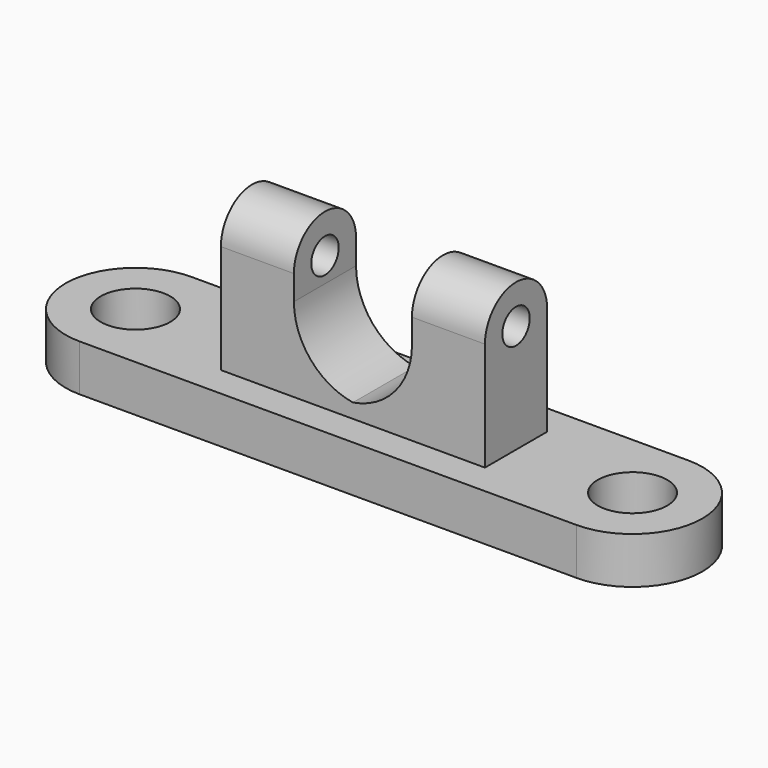
from build123d import *

# Parameters (mm, degrees)
F0_R        = 22.3974192725
F1_DEPTH    = 30
F2_W        = 85
F2_H        = 50
F3_DEPTH    = 70
F4_W        = 38
F4_H        = 60.7357084751
F5_DEPTH    = 50
F6_T1_DEPTH = 50
F8_DEPTH    = 47
F9_R        = 11.0426148683
F10_DEPTH   = 47


# Not quite as in the source:
# - a fillet or chamfer that OpenCascade refuses, or shapes differently, is made with other operations: its cross-section is extruded or revolved along the edge and cut away or added


with BuildPart() as f1:
    # F0 (on Top) → F1 (new body)
    with BuildSketch(Plane.XY):
        with BuildLine():
            Line((0, 0), (0, 45))
            Line((0, 45), (-160, 45))
            ThreePointArc((-160, 45), (-205, 0), (-160, -45))
            Line((-160, -45), (0, -45))
            Line((0, -45), (0, 0))
        make_face()
        with Locations((-160, 0)):
            Circle(F0_R, mode=Mode.SUBTRACT)
    extrude(amount=F1_DEPTH)

    # F2 (on face) → F3 (join)
    with BuildSketch(Plane.XY.offset(30)):
        with Locations((-42.5, 0)):
            Rectangle(F2_W, F2_H)
    extrude(amount=F3_DEPTH)

    # F4 (on face) → F5 (cut)
    with BuildSketch(Plane.XZ.offset(25)):
        with Locations((-19, 69.6321457624)):
            Rectangle(F4_W, F4_H)
    extrude(amount=-F5_DEPTH, mode=Mode.SUBTRACT)

    # F6: fillet of radius 45.3872149726 on 1 edges, made by hand

    # F6_s2 → F6_t1 (join)
    with BuildSketch(Plane.XZ.offset(-25)):
        with BuildLine():
            ThreePointArc((0, 39.2642915249), (-27.2197525121, 54.6803835575), (-38, 84.0463006125))
            Line((-38, 84.0463006125), (-38, 39.2642915249))
            Line((-38, 39.2642915249), (0, 39.2642915249))
        make_face()
    extrude(amount=F6_T1_DEPTH)

    # F7 (on face) → F8 (join)
    with BuildSketch(Plane(origin=(-85, 0, 0), x_dir=(0, -1, 0), z_dir=(-1, 0, 0))):
        with BuildLine():
            Line((-25, 100), (25, 100))
            ThreePointArc((25, 100), (0, 125), (-25, 100))
        make_face()
    extrude(amount=-F8_DEPTH)

    # F9 (on face) → F10 (cut)
    with BuildSketch(Plane(origin=(-85, 0, 0), x_dir=(0, -1, 0), z_dir=(-1, 0, 0))):
        with Locations((0, 100)):
            Circle(F9_R)
    extrude(amount=-F10_DEPTH, mode=Mode.SUBTRACT)

    # F11: F1 across face


with BuildPart() as f1_1:
    add(f1.part)
    add(f1.part.mirror(Plane(origin=(0, 0, 17.8748906724), x_dir=(0, 1, 0), z_dir=(1, 0, 0))))


solid = f1_1.part
